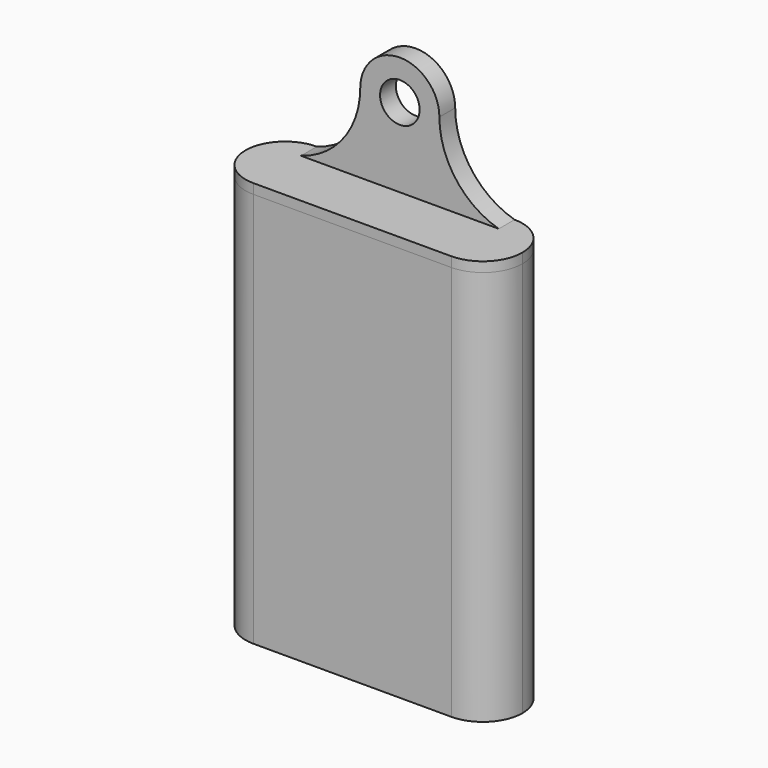
from build123d import *

# Parameters (mm, degrees)
F0_W      = 177.8
F0_H      = 50.8
F1_DEPTH  = 127
F2_R      = 25.39999
F3_W      = 101.6
F3_H      = 127
F3_W_2    = 50.8
F3_H_2    = 25.4
F4_DEPTH  = 12.7
F5_DEPTH  = 15.24
F6_DEPTH  = 15.24
F7_DEPTH  = 15.24
F8_DEPTH  = 12.7
F10_DEPTH = 50.8
F11_DEPTH = 12.7
F12_R     = 25.39999


# Not quite as in the source:
# - a fillet or chamfer is up to 0.001 mm smaller than in the source, because OpenCascade refuses the exact size
# - ends of sketch curves that miss each other by under 0.0002 mm in the source are joined


with BuildPart() as f1:
    # F0 (on Top) → F1 (new body, symmetric)
    with BuildSketch(Plane.XY):
        Rectangle(F0_W, F0_H)
    extrude(amount=F1_DEPTH, both=True)

    # F2 (radius 25.4 in the source; OpenCascade refuses exactly that, so slightly less here)
    f2_edges = [f1.edges().sort_by_distance(p)[0] for p in [
        (-88.9, -25.4, 0),
        (-88.9, 25.4, 0),
        (88.9, -25.4, 0),
        (88.9, 25.4, 0),
    ]]
    fillet(f2_edges, radius=F2_R)

    # F3 (on face) → F4 (cut)
    with BuildSketch(Plane(origin=(0, 25.4, 0), x_dir=(-1, 0, 0), z_dir=(0, 1, 0))):
        with Locations((0, 50.8)):
            Rectangle(F3_W, F3_H)
        with Locations((0, -88.9)):
            Rectangle(F3_W_2, F3_H_2)
        with BuildLine():
            Line((-38.1, -102.4676784873), (-38.1, -77.0676784873))
            ThreePointArc((-38.1, -77.0676784873), (-50.8, -89.7676784873), (-38.1, -102.4676784873))
        make_face()
        with BuildLine():
            ThreePointArc((38.1, -102.4676784873), (50.8, -89.7676784873), (38.1, -77.0676784873))
            Line((38.1, -77.0676784873), (38.1, -102.4676784873))
        make_face()
    extrude(amount=-F4_DEPTH, mode=Mode.SUBTRACT)


with BuildPart() as f5:
    # F5 (new): a face of the model
    f5_faces = [f1.part.faces().sort_by_distance(p)[0] for p in [
        (43.490047406, 12.7, -89.7676784873),
    ]]
    extrude(f5_faces, amount=F5_DEPTH)


with BuildPart() as f6:
    # F6 (new): a face of the model
    f6_faces = [f1.part.faces().sort_by_distance(p)[0] for p in [
        (0, 12.7, -88.9),
    ]]
    extrude(f6_faces, amount=F6_DEPTH)


with BuildPart() as f7:
    # F7 (new): a face of the model
    f7_faces = [f1.part.faces().sort_by_distance(p)[0] for p in [
        (-43.490047406, 12.7, -89.7676784873),
    ]]
    extrude(f7_faces, amount=F7_DEPTH)


with BuildPart() as f8:
    # F8 (new): a face of the model
    f8_faces = [f1.part.faces().sort_by_distance(p)[0] for p in [
        (0, 12.7, 50.8),
    ]]
    extrude(f8_faces, amount=F8_DEPTH)


with BuildPart() as f10:
    # F9 (on face) → F10 (new body)
    with BuildSketch(Plane(origin=(0, 25.4, 0), x_dir=(-1, 0, 0), z_dir=(0, 1, 0))):
        Polygon((-88.9, 127), (-63.5000066667, 127), (63.5, 127), (88.9, 127), (88.9, 133.35), (63.5, 133.35), (25.4, 133.35), (-25.4, 133.35), (-63.5, 133.35), (-88.9, 133.35), align=None)
    extrude(amount=-F10_DEPTH)

    # F9 (on face) → F11 (join)
    with BuildSketch(Plane(origin=(0, 25.4, 0), x_dir=(-1, 0, 0), z_dir=(0, 1, 0))):
        with BuildLine():
            Line((-25.4, 184.15), (-25.4, 133.35))
            Line((-25.4, 133.35), (25.4, 133.35))
            Line((25.4, 133.35), (25.4, 184.15))
            Line((25.4, 184.15), (12.7, 184.15))
            ThreePointArc((12.7, 184.15), (0, 171.45), (-12.7, 184.15))
            Line((-12.7, 184.15), (-25.4, 184.15))
        make_face()
        with BuildLine():
            Line((25.4, 133.35), (63.5, 133.35))
            ThreePointArc((63.5, 133.35), (35.9833333333, 152.4), (25.4, 184.15))
            Line((25.4, 184.15), (25.4, 133.35))
        make_face()
        with BuildLine():
            ThreePointArc((-25.4, 184.15), (-35.9833333333, 152.4), (-63.5, 133.35))
            Line((-63.5, 133.35), (-25.4, 133.35))
            Line((-25.4, 133.35), (-25.4, 184.15))
        make_face()
        with BuildLine():
            ThreePointArc((25.4, 184.15), (0, 209.55), (-25.4, 184.15))
            Line((-25.4, 184.15), (-12.7, 184.15))
            ThreePointArc((-12.7, 184.15), (0, 196.85), (12.7, 184.15))
            Line((12.7, 184.15), (25.4, 184.15))
        make_face()
    extrude(amount=-F11_DEPTH)

    # F12 (radius 25.4 in the source; OpenCascade refuses exactly that, so slightly less here)
    f12_edges = [f10.edges().sort_by_distance(p)[0] for p in [
        (-88.9, -25.4, 130.175),
        (-88.9, 25.4, 130.175),
        (88.9, -25.4, 130.175),
        (88.9, 25.4, 130.175),
    ]]
    fillet(f12_edges, radius=F12_R)


solid = Compound([f1.part, f5.part, f6.part, f7.part, f8.part, f10.part])
